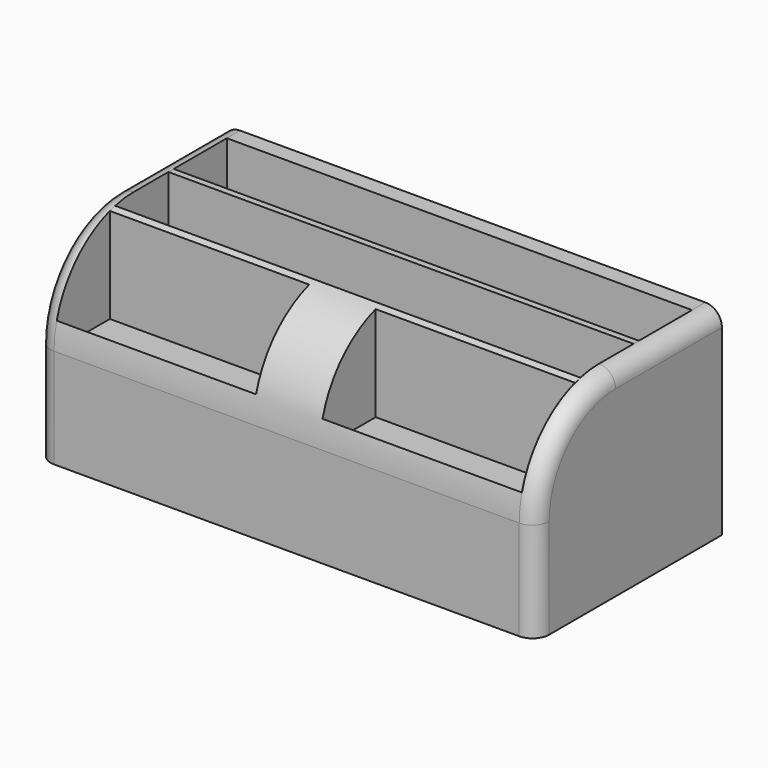
from build123d import *

# Parameters (mm, degrees)
F0_W        = 150
F0_H        = 70
F0_W_2      = 60
F0_H_2      = 20
F0_W_3      = 140
F1_DEPTH    = 60
F2_T1_DEPTH = 300
F3_R        = 4.99999
F4_W        = 140
F4_H        = 20.1229466498
F4_H_2      = 20
F5_DEPTH    = 30


# Not quite as in the source:
# - a fillet or chamfer that OpenCascade refuses, or shapes differently, is made with other operations: its cross-section is extruded or revolved along the edge and cut away or added
# - a fillet or chamfer is up to 0.001 mm smaller than in the source, because OpenCascade refuses the exact size


with BuildPart() as f1:
    # F0 (on Top) → F1 (new body)
    with BuildSketch(Plane.XY):
        Rectangle(F0_W, F0_H)
        with Locations((-40, -24)):
            Rectangle(F0_W_2, F0_H_2, mode=Mode.SUBTRACT)
        with Locations((40, -24)):
            Rectangle(F0_W_2, F0_H_2, mode=Mode.SUBTRACT)
        with Locations((0, -2)):
            Rectangle(F0_W_3, F0_H_2, mode=Mode.SUBTRACT)
        with Locations((0, 20)):
            Rectangle(F0_W_3, F0_H_2, mode=Mode.SUBTRACT)
    extrude(amount=F1_DEPTH)

    # F2: fillet of radius 30 on 1 edges, made by hand

    # F2_s2 → F2_t1 (cut)
    with BuildSketch(Plane.YZ.offset(-150)):
        with BuildLine():
            ThreePointArc((-35, 30), (-26.2132034356, 51.2132034356), (-5, 60))
            Line((-5, 60), (-35, 60))
            Line((-35, 60), (-35, 30))
        make_face()
    extrude(amount=F2_T1_DEPTH, mode=Mode.SUBTRACT)

    # F3 (radius 5 in the source; OpenCascade refuses exactly that, so slightly less here)
    f3_edges = [f1.edges().sort_by_distance(p)[0] for p in [
        (75, 15, 60),
        (-75, 15, 60),
    ]]
    fillet(f3_edges, radius=F3_R)

    # F4 (on face) → F5 (join)
    with BuildSketch(Plane(origin=(0, 0, 0), x_dir=(1, 0, 0), z_dir=(0, 0, -1))):
        with Locations((0, -19.9385266751)):
            Rectangle(F4_W, F4_H)
        with Locations((0, 2)):
            Rectangle(F4_W, F4_H_2)
        with Locations((0, 24)):
            Rectangle(F4_W, F4_H_2)
    extrude(amount=-F5_DEPTH)


solid = f1.part
